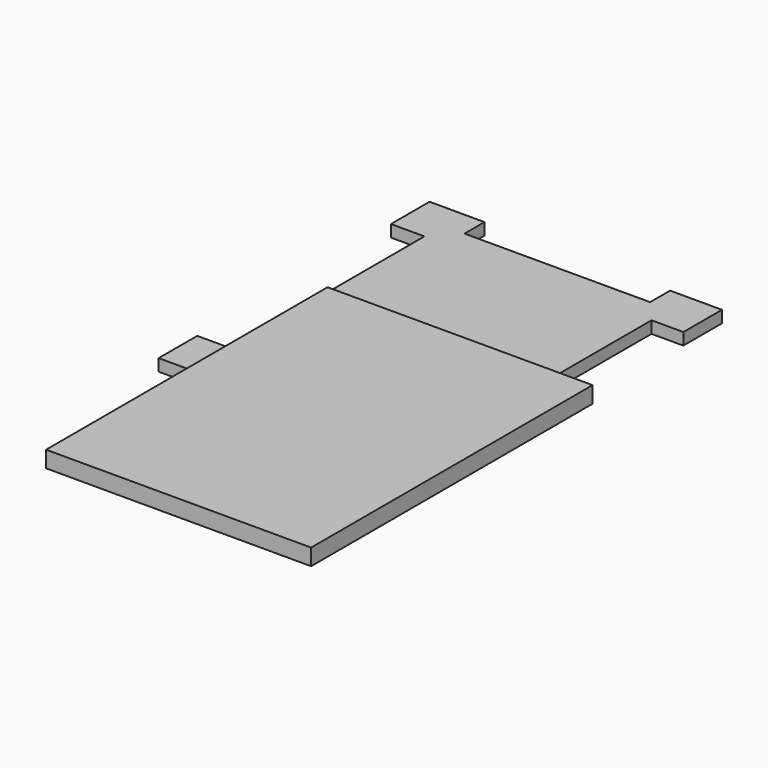
from build123d import *

# Parameters (mm, degrees)
F0_W     = 48.3713261783
F0_H     = 64.2076134682
F1_DEPTH = 3
F0_W_2   = 12.6881040633
F0_H_2   = 12.7290943637
F4_W     = 3.9221420884
F4_H     = 4.2427778244
F4_W_2   = 3.6538615823
F5_DEPTH = 2.1847370081


with BuildPart() as f1:
    # F0 (on Top) → F1 (new body)
    with BuildSketch(Plane.XY):
        with Locations((24.1856630892, -32.1038067341)):
            Rectangle(F0_W, F0_H)
    extrude(amount=F1_DEPTH)


with BuildPart() as f1b:
    # F0 (on Top) → F1, piece 2 (new body)
    with BuildSketch(Plane.XY):
        Polygon((60.9453171492, -64.2076134682), (48.3713261783, -64.2076134682), (48.8873720169, -77.1873742342), (60.9453171492, -77.1873742342), align=None)
    extrude(amount=F1_DEPTH)


with BuildPart() as f1c:
    # F0 (on Top) → F1, piece 3 (new body)
    with BuildSketch(Plane.XY):
        with Locations((54.7153782099, 6.3645471819)):
            Rectangle(F0_W_2, F0_H_2)
    extrude(amount=F1_DEPTH)


with BuildPart() as f5:
    # F4 (on Top) → F5 (new body)
    with BuildSketch(Plane.XY):
        Polygon((0, 22.0977440476), (0, 0), (41.4505898952, 0), (41.4505898952, 22.0977440476), (37.796728313, 22.0977440476), (37.796728313, 26.340521872), (3.9221420884, 26.340521872), (3.9221420884, 22.0977440476), align=None)
        Polygon((-6.1037912965, 22.0977440476), (0, 22.0977440476), (0, 26.340521872), (3.9221420884, 26.340521872), (3.9221420884, 30.8983102441), (-6.1037912965, 30.8983102441), align=None)
        with Locations((1.9610710442, 24.2191329598)):
            Rectangle(F4_W, F4_H)
        with Locations((39.6236591041, 24.2191329598)):
            Rectangle(F4_W_2, F4_H)
        Polygon((41.4505898952, 26.340521872), (41.4505898952, 22.0977440476), (47.2597032785, 22.0977440476), (47.2597032785, 30.8983102441), (37.796728313, 30.8983102441), (37.796728313, 26.340521872), align=None)
    extrude(amount=F5_DEPTH)

    # F8: F5 across plane


with BuildPart() as f5_1:
    add(f5.part)
    add(f5.part.mirror(Plane.XZ))


solid = Compound([f1.part, f5_1.part])
